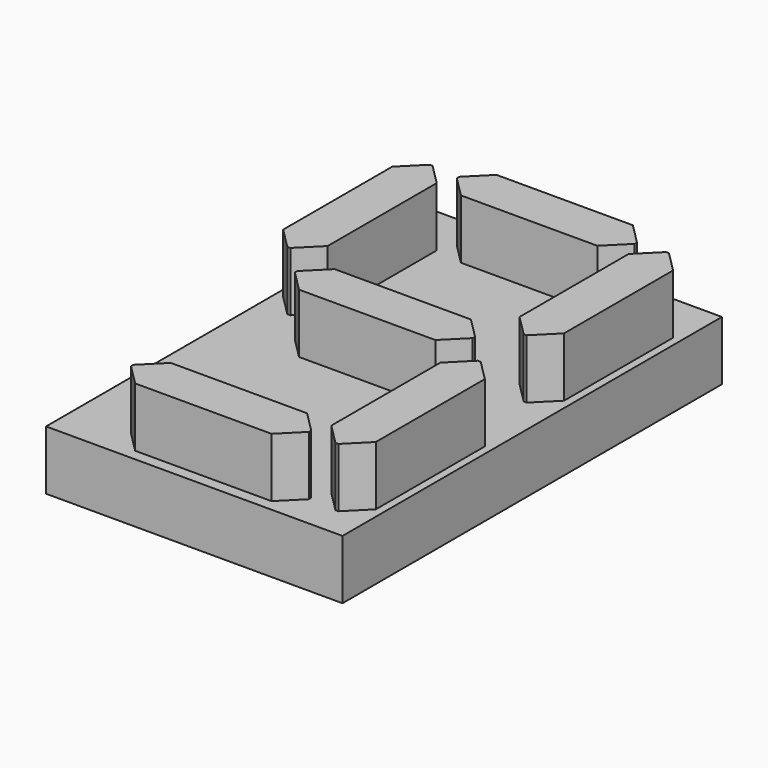
from build123d import *

# Parameters (mm, degrees)
F0_W     = 10
F0_H     = 16
F1_DEPTH = 2
F2_W     = 1.5
F2_H     = 6
F2_W_2   = 6
F2_H_2   = 1.5
F3_DEPTH = 2
F4_SIZE  = 0.7


# Not quite as in the source:
# - a feature names something its author has since deleted; it is built from what else it names


with BuildPart() as f1:
    # F0 (on Top) → F1 (new body)
    with BuildSketch(Plane.XY):
        Rectangle(F0_W, F0_H)
    extrude(amount=-F1_DEPTH)

    # F2 (on face) → F3 (join)
    with BuildSketch(Plane.XY):
        with Locations((-3.9874258153, 3.9691079506)):
            Rectangle(F2_W, F2_H)
        with Locations((0, 6.8687610328)):
            Rectangle(F2_W_2, F2_H_2)
        with Locations((3.9874258153, 3.9691079506)):
            Rectangle(F2_W, F2_H)
        with Locations((0.0284713751, 0.0055548735)):
            Rectangle(F2_W_2, F2_H_2)
        with Locations((0, -6.8687610328)):
            Rectangle(F2_W_2, F2_H_2)
        with Locations((3.9874258153, -3.9691079506)):
            Rectangle(F2_W, F2_H)
    extrude(amount=F3_DEPTH)

    # F4
    f4_edges = [f1.edges().sort_by_distance(p)[0] for p in [
        (3, 6.118761, 1),
        (3.237426, 6.969108, 1),
        (3.237426, 0.969108, 1),
        (4.737426, 0.969108, 1),
        (3.237426, -0.969108, 1),
        (3.028471, -0.744445, 1),
        (-2.971529, -0.744445, 1),
        (-2.971529, 0.755555, 1),
        (-3.237426, 0.969108, 1),
        (-4.737426, 0.969108, 1),
        (-4.737426, 6.969108, 1),
        (-3, 6.118761, 1),
        (-3, 7.618761, 1),
        (3.237426, -6.969108, 1),
        (4.737426, -6.969108, 1),
        (3, -7.618761, 1),
        (-3, -7.618761, 1),
        (-3, -6.118761, 1),
        (3.028471, 0.755555, 1),
        (4.737426, -0.969108, 1),
        (3, -6.118761, 1),
        (4.737426, 6.969108, 1),
        (3, 7.618761, 1),
        (-3.237426, 6.969108, 1),
    ]]
    chamfer(f4_edges, length=F4_SIZE)


solid = f1.part
